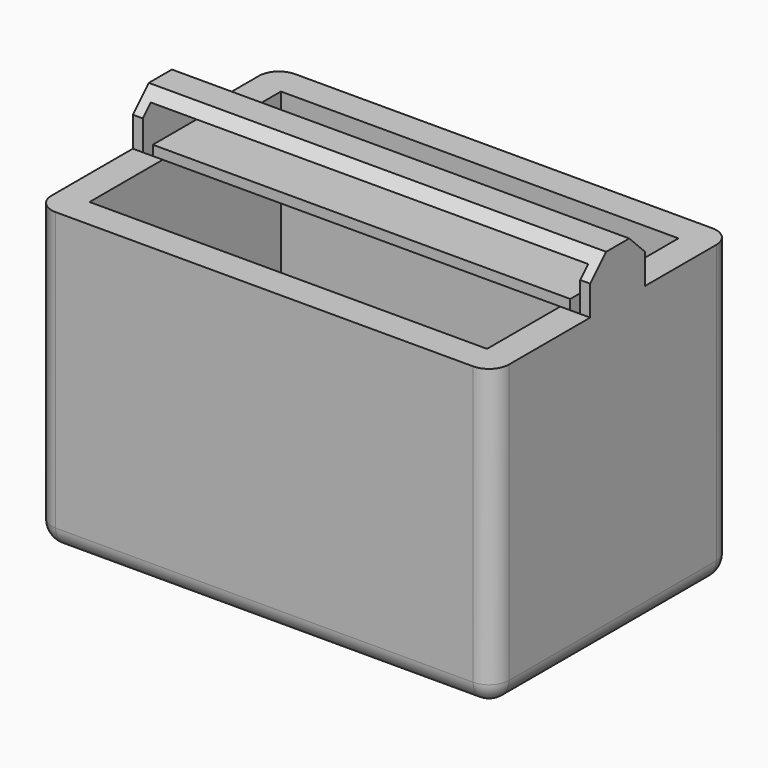
from build123d import *

# Parameters (mm, degrees)
F0_W         = 116.5109202266
F0_H         = 75.9218987077
F1_DEPTH     = 76.2
F2_T         = -7.62
F3_W         = 116.5109202266
F3_H         = 17.5204388797
F4_DEPTH     = 12.7
F5_T         = -2.54
F6_R         = 5.08
F7_R         = 5.08
F8_R         = 5.08
F9_T1_DEPTH  = 66.04
F9_T3_DEPTH  = 106.3509202266
F9_T5_DEPTH  = 83.5418987077
F9_S9_W      = 5.08
F9_S9_H      = 5.08
F9_T10_DEPTH = 5.08
F9_T14_ANGLE = 90
F9_T16_ANGLE = 90
F10_T1_DEPTH = 142.6392193843
F11_T1_DEPTH = 142.6392193843


# Not quite as in the source:
# - a fillet or chamfer that OpenCascade refuses, or shapes differently, is made with other operations: its cross-section is extruded or revolved along the edge and cut away or added
# - a shell that OpenCascade refuses in one call is made with other operations: the cavity is built on its own and cut out


with BuildPart() as f1:
    # F0 (on Front) → F1 (new body)
    with BuildSketch(Plane.XZ):
        with Locations((6.8621747196, 17.2284292057)):
            Rectangle(F0_W, F0_H)
    extrude(amount=F1_DEPTH)

    # F2
    f2_openings = [f1.faces().sort_by_distance(p)[0] for p in [
        (6.862175, -38.1, 55.189379),
    ]]
    offset(amount=F2_T, openings=f2_openings)

    # F3 (on face) → F4 (join)
    with BuildSketch(Plane.XY.offset(55.1893785596)):
        with Locations((6.8621747196, -36.5009140223)):
            Rectangle(F3_W, F3_H)
    extrude(amount=F4_DEPTH)

    # F5: a shell. OpenCascade refuses it in one call, so the cavity is built on its own and cut out:
    # the body offset inwards by the wall thickness, plus a prism from it out through each open face.
    f5_core = offset(f1.part, amount=F5_T, kind=Kind.INTERSECTION, mode=Mode.PRIVATE)
    f5_exits = [f5_core.faces().sort_by_distance(p)[0] for p in [
        (6.862175, -42.721133, 61.352079),
        (6.862175, -30.280695, 61.352079),
    ]]
    add(f5_core, mode=Mode.SUBTRACT)
    extrude(f5_exits, amount=-F5_T, mode=Mode.SUBTRACT)

    # F6
    f6_edges = [f1.edges().sort_by_distance(p)[0] for p in [
        (65.117635, 0, 17.228429),
    ]]
    fillet(f6_edges, radius=F6_R)

    # F7
    f7_edges = [f1.edges().sort_by_distance(p)[0] for p in [
        (4.322175, 0, -20.73252),
        (-51.393285, 0, 17.228429),
    ]]
    fillet(f7_edges, radius=F7_R)

    # F8
    f8_edges = [f1.edges().sort_by_distance(p)[0] for p in [
        (-51.393285, -76.2, 17.228429),
    ]]
    fillet(f8_edges, radius=F8_R)

    # F9: fillet of radius 5.08 on 1 edges, made by hand

    # F9_s2 → F9_t1 (cut)
    with BuildSketch(Plane.XZ.offset(5.08)):
        with BuildLine():
            ThreePointArc((-51.3932853937, -15.6525201482), (-49.9053878421, -19.2446225966), (-46.3132853937, -20.7325201482))
            Line((-46.3132853937, -20.7325201482), (-51.3932853937, -20.7325201482))
            Line((-51.3932853937, -20.7325201482), (-51.3932853937, -15.6525201482))
        make_face()
    extrude(amount=F9_T1_DEPTH, mode=Mode.SUBTRACT)

    # F9_s4 → F9_t3 (cut)
    with BuildSketch(Plane.YZ.offset(-46.3132853937)):
        with BuildLine():
            ThreePointArc((-71.12, -20.7325201482), (-74.7121024484, -19.2446225966), (-76.2, -15.6525201482))
            Line((-76.2, -15.6525201482), (-76.2, -20.7325201482))
            Line((-76.2, -20.7325201482), (-71.12, -20.7325201482))
        make_face()
    extrude(amount=F9_T3_DEPTH, mode=Mode.SUBTRACT)

    # F9_s6 → F9_t5 (cut)
    with BuildSketch(Plane.XY.offset(-15.6525201482)):
        with BuildLine():
            ThreePointArc((60.0376348329, -76.2), (63.6297372813, -74.7121024484), (65.1176348329, -71.12))
            Line((65.1176348329, -71.12), (65.1176348329, -76.2))
            Line((65.1176348329, -76.2), (60.0376348329, -76.2))
        make_face()
    extrude(amount=F9_T5_DEPTH, mode=Mode.SUBTRACT)


with BuildPart() as f9_tool8:
    # F9_s9 → F9_t10 (new body)
    with BuildSketch(Plane.YZ.offset(-46.3132853937)):
        with Locations((-2.54, -18.1925201482)):
            Rectangle(F9_S9_W, F9_S9_H)
    extrude(amount=-F9_T10_DEPTH)

    # F9_s11 → F9_t12 (revolve, cut)
    with BuildSketch(Plane(origin=(-46.3132853937, -5.08, -15.6525201482), x_dir=(0, -0.7071067812, 0.7071067812), z_dir=(0, -0.7071067812, -0.7071067812))):
        with BuildLine():
            ThreePointArc((0, -5.08), (5.08, 0), (0, 5.08))
            Line((0, 5.08), (0, -5.08))
        make_face()
    revolve(axis=Axis((-46.3132853937, -5.08, -15.6525201482), (-1, 0, 0)), mode=Mode.SUBTRACT)


with BuildPart() as f1_1:
    add(f1.part)

    # F9_t7: cut F9_tool8
    add(f9_tool8.part, mode=Mode.SUBTRACT)

    # F9_s13 → F9_t14 (revolve, cut)
    with BuildSketch(Plane.XZ.offset(71.12)):
        with BuildLine():
            ThreePointArc((-46.3132853937, -20.7325201482), (-49.9053878421, -19.2446225966), (-51.3932853937, -15.6525201482))
            Line((-51.3932853937, -15.6525201482), (-51.3932853937, -20.7325201482))
            Line((-51.3932853937, -20.7325201482), (-46.3132853937, -20.7325201482))
        make_face()
    revolve(axis=Axis((-46.3132853937, -71.12, -20.7325201482), (0, 0, 1)), revolution_arc=F9_T14_ANGLE, mode=Mode.SUBTRACT)

    # F9_s15 → F9_t16 (revolve, cut)
    with BuildSketch(Plane.XY.offset(-15.6525201482)):
        with BuildLine():
            ThreePointArc((60.0376348329, -76.2), (63.6297372813, -74.7121024484), (65.1176348329, -71.12))
            Line((65.1176348329, -71.12), (65.1176348329, -76.2))
            Line((65.1176348329, -76.2), (60.0376348329, -76.2))
        make_face()
    revolve(axis=Axis((60.0376348329, -76.2, -15.6525201482), (0, 1, 0)), revolution_arc=F9_T16_ANGLE, mode=Mode.SUBTRACT)

    # F10: chamfer of 5.08 on 1 edges, made by hand

    # F10_s2 → F10_t1 (cut)
    with BuildSketch(Plane.YZ.offset(-64.4574349726)):
        Polygon((-45.2611334622, 62.8093785596), (-40.1811334622, 67.8893785596), (-45.2611334622, 67.8893785596), align=None)
    extrude(amount=F10_T1_DEPTH, mode=Mode.SUBTRACT)

    # F11: chamfer of 5.08 on 1 edges, made by hand

    # F11_s2 → F11_t1 (cut)
    with BuildSketch(Plane.YZ.offset(-64.4574349726)):
        Polygon((-32.8206945825, 67.8893785596), (-27.7406945825, 62.8093785596), (-27.7406945825, 67.8893785596), align=None)
    extrude(amount=F11_T1_DEPTH, mode=Mode.SUBTRACT)


solid = f1_1.part
